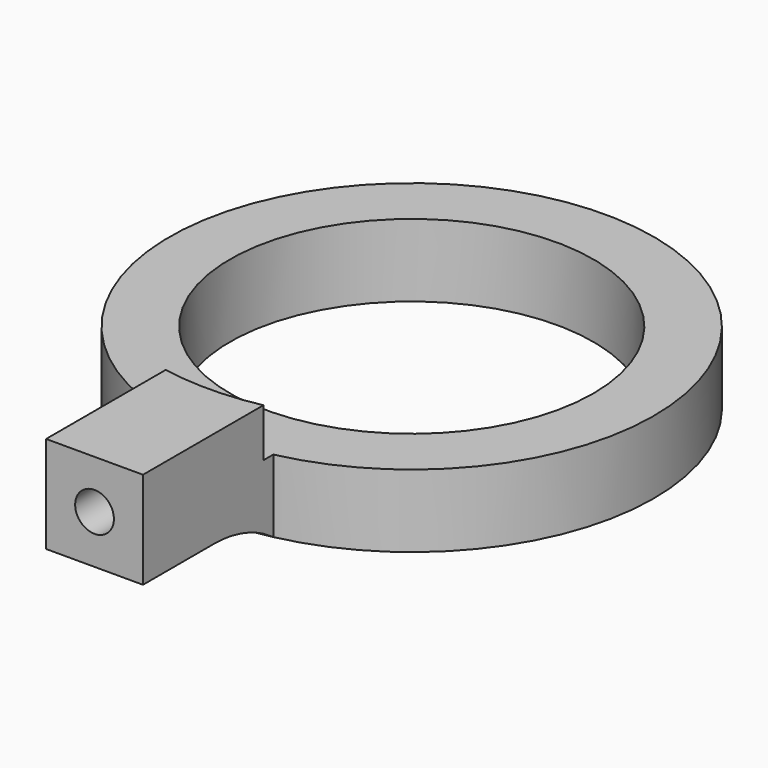
from build123d import *

# Parameters (mm, degrees)
F0_R        = 10
F0_R_2      = 7.5
F1_DEPTH    = 3
F3_W        = 4
F3_H        = 7
F4_DEPTH    = 4
F5_R        = 10.5
F6_DEPTH    = 25
F7_T4_ANGLE = 109.021242163
F9_D        = 1.6
F9_DEPTH    = 6
F9_TIP      = 0.4806884952


# Not quite as in the source:
# - a fillet or chamfer that OpenCascade refuses, or shapes differently, is made with other operations: its cross-section is extruded or revolved along the edge and cut away or added


with BuildPart() as f1:
    # F0 (on Top) → F1 (new body)
    with BuildSketch(Plane.XY):
        Circle(F0_R)
        Circle(F0_R_2, mode=Mode.SUBTRACT)
    extrude(amount=F1_DEPTH)

    # F3 (on offset) → F4 (join)
    with BuildSketch(Plane.XY.offset(1)):
        with Locations((0.106652909, -13)):
            Rectangle(F3_W, F3_H)
    extrude(amount=F4_DEPTH)

    # F5 (on face) → F6 (cut)
    with BuildSketch(Plane.XY.offset(3)):
        Circle(F5_R)
    extrude(amount=F6_DEPTH, mode=Mode.SUBTRACT)

    # F7: fillet of radius 5 on 1 edges, made by hand


with BuildPart() as f7_tool2:
    # F7_s3 → F7_t4 (revolve)
    with BuildSketch(Plane(origin=(0, 0, 0), x_dir=(0, 0, 1), z_dir=(0.5716546179, 0.8204943618, 0))):
        with BuildLine():
            ThreePointArc((0, 10), (0.7434164903, 11.4188611699), (1, 13))
            Line((1, 13), (1, 10))
            Line((1, 10), (0, 10))
        make_face()
    revolve(axis=Axis((0, 0, 1), (0, 0, -1)), revolution_arc=F7_T4_ANGLE)

    split(bisect_by=Plane.YZ.offset(2.106652909), keep=Keep.BOTTOM)

    split(bisect_by=Plane.YZ.offset(-1.893347091), keep=Keep.TOP)


with BuildPart() as f1_1:
    add(f1.part)

    # F7_t1: union F7_tool2
    add(f7_tool2.part)

    # F9
    with Locations(Plane.XZ.offset(16.5)):
        with Locations((0.106652909, 3)):
            Hole(F9_D / 2, depth=F9_DEPTH)
            with Locations((0, 0, -(F9_DEPTH + F9_TIP / 2))):  # 118° drill point
                Cone(0, F9_D / 2, F9_TIP, mode=Mode.SUBTRACT)


solid = f1_1.part
